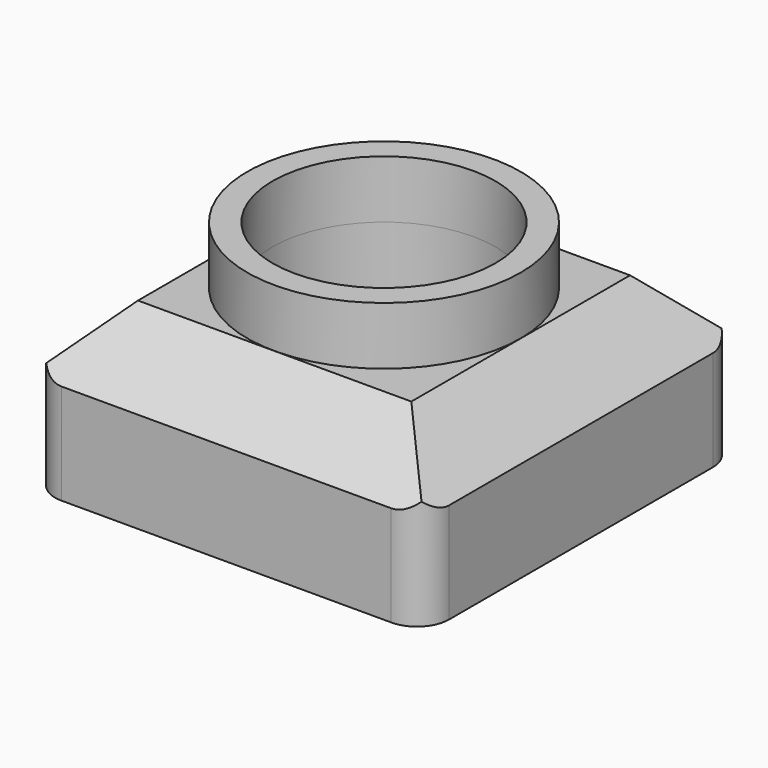
from build123d import *

# Parameters (mm, degrees)
F0_W     = 24.5
F0_H     = 24.5
F0_R     = 8.5
F0_R_2   = 6.925
F1_DEPTH = 10
F2_DEPTH = 3.6
F3_DEPTH = 25
F4_SIZE2 = 3.74999
F4_SIZE  = 3.74999
F5_R     = 2


# Not quite as in the source:
# - a fillet or chamfer is up to 0.001 mm smaller than in the source, because OpenCascade refuses the exact size


with BuildPart() as f1:
    # F0 (on Top) → F1 (new body)
    with BuildSketch(Plane.XY):
        Rectangle(F0_W, F0_H)
        Circle(F0_R, mode=Mode.SUBTRACT)
        Circle(F0_R)
        Circle(F0_R_2, mode=Mode.SUBTRACT)
        Circle(F0_R_2)
    extrude(amount=-F1_DEPTH)

    # F0 (on Top) → F2 (join)
    with BuildSketch(Plane.XY):
        Circle(F0_R)
        Circle(F0_R_2, mode=Mode.SUBTRACT)
    extrude(amount=F2_DEPTH)

    # F0 (on Top) → F3 (cut)
    with BuildSketch(Plane.XY):
        Circle(F0_R_2)
    extrude(amount=-F3_DEPTH, mode=Mode.SUBTRACT)

    # F4 (size 3.75 and 3.75 in the source; OpenCascade refuses exactly that, so slightly less here)
    f4_edges = [f1.edges().sort_by_distance(p)[0] for p in [
        (0, -12.25, 0),
        (12.25, 0, 0),
        (0, 12.25, 0),
        (-12.25, 0, 0),
    ]]
    chamfer(f4_edges, length=F4_SIZE, length2=F4_SIZE2)

    # F5
    f5_edges = [f1.edges().sort_by_distance(p)[0] for p in [
        (12.25, -12.25, -6.874995),
        (12.25, 12.25, -6.874995),
        (-12.25, 12.25, -6.874995),
        (-12.25, -12.25, -6.874995),
    ]]
    fillet(f5_edges, radius=F5_R)


solid = f1.part
